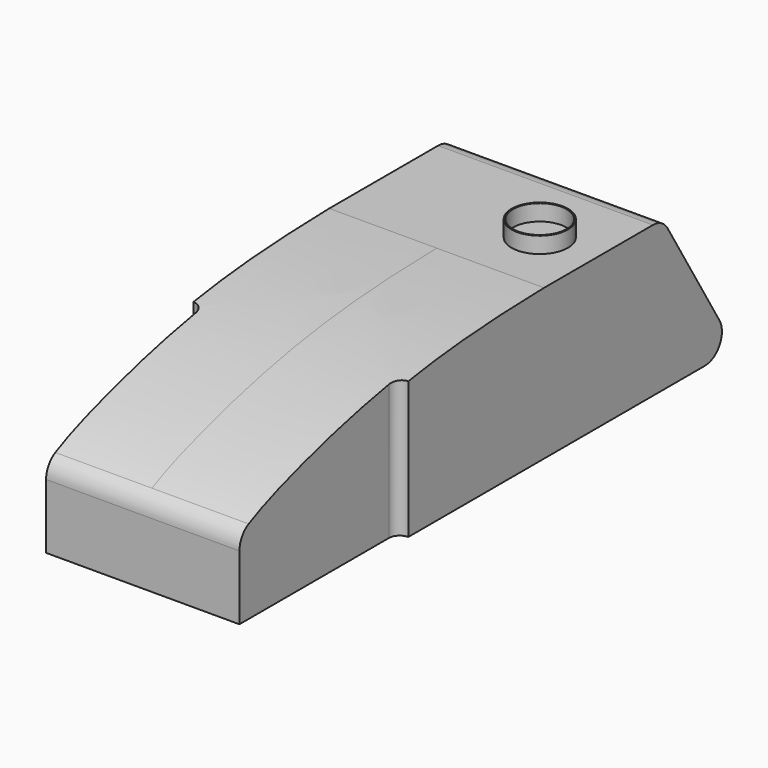
from build123d import *

# Parameters (mm, degrees)
F1_DEPTH = 127
F3_DEPTH = 177.8
F4_R     = 33.3375
F4_R_2   = 31.75
F5_DEPTH = 19.05
F6_T     = 7.62


# Not quite as in the source:
# - a shell that OpenCascade refuses in one call is made with other operations: the cavity is built on its own and cut out


with BuildPart() as f1:
    # F0 (on Right) → F1 (new body, symmetric)
    with BuildSketch(Plane.YZ):
        with BuildLine():
            Line((0, 76.4100525974), (0, 0))
            Line((0, 0), (671.8020987012, 0))
            ThreePointArc((671.8020987012, 0), (693.9200398628, 12.9117383606), (693.5512826501, 38.5199465532))
            Line((693.5512826501, 38.5199465532), (616.9399846733, 165.5199465532))
            ThreePointArc((616.9399846733, 165.5199465532), (607.6790623638, 174.5179411616), (595.1908007244, 177.8))
            Line((595.1908007244, 177.8), (434.3242754471, 177.8))
            add(Edge.make_bspline(
                [(434.3242754471, 177.8), (377.1008998353, 176.660223353), (237.5491375806, 169.4148859291), (92.7331109855, 131.2042560006), (30.2962614107, 107.6098996029), (13.6550616577, 98.9315184319)],
                knots=[0.1901896549, 0.1901896549, 0.1901896549, 0.1901896549, 0.3812653252, 0.674687688, 0.8202345165, 0.8202345165, 0.8202345165, 0.8202345165], degree=3))
            ThreePointArc((13.6550616577, 98.9315184319), (3.6804070723, 89.5789281398), (0, 76.4100525974))
        make_face()
    extrude(amount=F1_DEPTH, both=True)

    # F2 (on Top) → F3 (cut)
    with BuildSketch(Plane.XY):
        with BuildLine():
            Line((-127, 0), (-114.3, 0))
            Line((-114.3, 0), (-114.3, 220.98))
            ThreePointArc((-114.3, 220.98), (-118.0197438789, 229.9602561211), (-127, 233.68))
            Line((-127, 233.68), (-127, 0))
        make_face()
        with BuildLine():
            Line((114.3, 220.98), (114.3, 0))
            Line((114.3, 0), (127, 0))
            Line((127, 0), (127, 233.68))
            ThreePointArc((127, 233.68), (118.0197438789, 229.9602561211), (114.3, 220.98))
        make_face()
    extrude(amount=F3_DEPTH, mode=Mode.SUBTRACT)

    # F4 (on face) → F5 (join)
    with BuildSketch(Plane.XY.offset(177.8)):
        with Locations((60.96, 510.5242754471)):
            Circle(F4_R)
        with Locations((60.96, 510.5242754471)):
            Circle(F4_R_2, mode=Mode.SUBTRACT)
    extrude(amount=F5_DEPTH)

    # F6: shell of thickness 7.62, made by hand


with BuildPart() as f6_core1:
    # F6_t2: copy of F1
    add(f1.part)

    # the walls: a layer under each face that stays
    f6_faces = [f6_core1.faces().sort_by_distance(p)[0] for p in [
        (-63.5, 178.8934164203, 151.6082143397),
        (63.5, 178.8934164203, 151.6082143397),
        (0, 3.6804070723, 89.5789281398),
        (-114.3, 110.49, 79.9601525115),
        (-118.0197438789, 229.9602561211, 81.0374425071),
        (-127, 465.4410493506, 88.9),
        (0, 514.7575380857, 177.8),
        (114.3, 110.49, 79.9601525115),
        (118.0197438789, 229.9602561211, 81.0374425071),
        (127, 465.4410493506, 88.9),
        (0, 0, 38.2050262987),
        (0, 607.6790623638, 174.5179411616),
        (0, 655.2456336617, 102.0199465532),
        (0, 693.9200398628, 12.9117383606),
        (27.6225, 510.5242754471, 187.325),
        (29.845, 501.6342754471, 196.85),
        (29.21, 510.5242754471, 187.325),
        (60.96, 510.5242754471, 177.8),
    ]]
    thicken(f6_faces, amount=-F6_T, mode=Mode.SUBTRACT)

    # F6_s3 → F6_t4 (revolve, cut)
    with BuildSketch(Plane.XZ.offset(-510.5242754471)):
        Polygon((94.3737, 177.8762), (94.2975, 170.18), (86.6775, 170.18), (86.6775, 177.8), align=None)
    revolve(axis=Axis((60.96, 510.5242754471, 177.8), (0, 0, 1)), mode=Mode.SUBTRACT)

    # F6_s5 → F6_t6 (revolve, cut)
    with BuildSketch(Plane.XZ.offset(-510.5242754471)):
        Polygon((92.6338, 177.8762), (100.33, 177.8), (100.33, 170.18), (92.71, 170.18), align=None)
    revolve(axis=Axis((60.96, 510.5242754471, 177.8), (0, 0, 1)), mode=Mode.SUBTRACT)


with BuildPart() as f1_1:
    add(f1.part)

    # what is left inside the walls is the cavity
    f6_cavity = [f6_core1.part.solids().sort_by_distance(p)[0] for p in [
        (-39.793333, 339.711049, 0.0762),
    ]]
    add(f6_cavity, mode=Mode.SUBTRACT)


solid = f1_1.part
